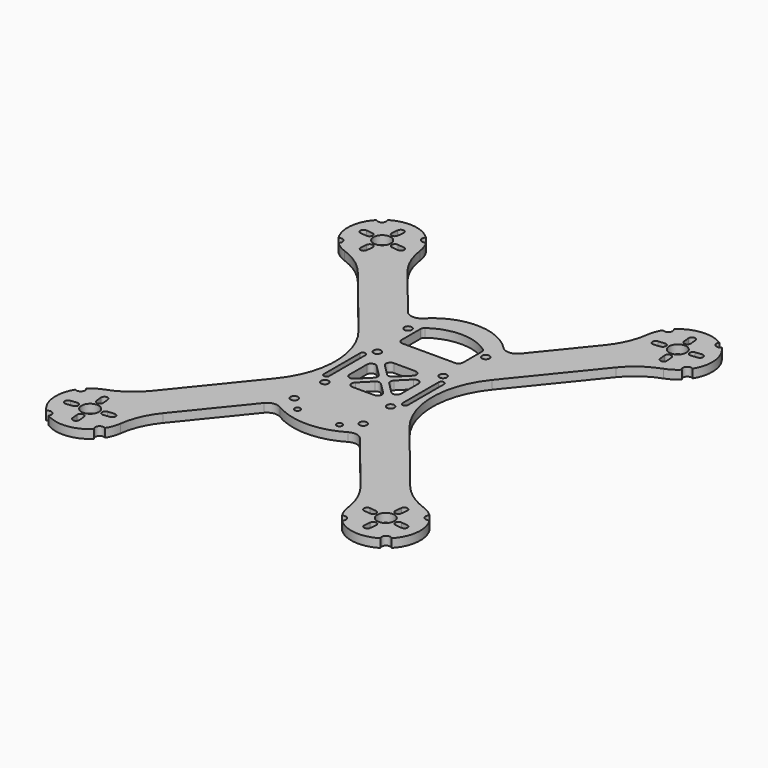
from build123d import *

# Parameters (mm, degrees)
F0_R     = 4
F0_R_2   = 1.35
F0_R_3   = 1.75
F1_DEPTH = 4
F3_DEPTH = 25


# Not quite as in the source:
# - a feature names something its author has since deleted; it is built from what else it names


with BuildPart() as f1:
    # F0 (on Top) → F1 (new body)
    with BuildSketch(Plane.XY):
        with BuildLine():
            ThreePointArc((59.8824194875, 59.6474879899), (66.2441988356, 65.6146941014), (73.980978501, 69.6423516913))
            ThreePointArc((73.980978501, 69.6423516913), (77.0154819314, 71.1033586862), (79.6769346686, 73.1671953648))
            ThreePointArc((79.6769346686, 73.1671953648), (79.4759660848, 75.8984243241), (82.1892948565, 76.269701817))
            ThreePointArc((82.1892948565, 76.269701817), (84.5082729503, 86.3813652111), (80.1376370585, 95.789921843))
            ThreePointArc((80.1376370585, 95.789921843), (77.4064080991, 95.5889532592), (77.0351306062, 98.3022820309))
            ThreePointArc((77.0351306062, 98.3022820309), (66.9234672121, 100.6212601247), (57.5149105803, 96.2506242328))
            ThreePointArc((57.5149105803, 96.2506242328), (57.715879164, 93.5193952735), (55.0025503923, 93.1481177806))
            ThreePointArc((55.0025503923, 93.1481177806), (53.5371606356, 90.1157283978), (52.7389888878, 86.8437757133))
            ThreePointArc((52.7389888878, 86.8437757133), (50.4079122214, 78.4386661467), (45.8937921813, 70.9752550288))
            Line((45.8937921813, 70.9752550288), (26.0751424851, 46.5012608726))
            ThreePointArc((26.0751424851, 46.5012608726), (22.420247462, 44.6531941399), (18.6104751491, 46.1562720492))
            ThreePointArc((18.6104751491, 46.1562720492), (0, 54), (-18.6104751491, 46.1562720492))
            ThreePointArc((-18.6104751491, 46.1562720492), (-22.420247462, 44.6531941399), (-26.0751424851, 46.5012608726))
            Line((-26.0751424851, 46.5012608726), (-45.8937921813, 70.9752550288))
            ThreePointArc((-45.8937921813, 70.9752550288), (-50.4079122214, 78.4386661467), (-52.7389888878, 86.8437757133))
            ThreePointArc((-52.7389888878, 86.8437757133), (-53.5371606356, 90.1157283978), (-55.0025503923, 93.1481177806))
            ThreePointArc((-55.0025503923, 93.1481177806), (-57.715879164, 93.5193952735), (-57.5149105803, 96.2506242328))
            ThreePointArc((-57.5149105803, 96.2506242328), (-66.9234672121, 100.6212601247), (-77.0351306062, 98.3022820309))
            ThreePointArc((-77.0351306062, 98.3022820309), (-77.4064080991, 95.5889532592), (-80.1376370585, 95.789921843))
            ThreePointArc((-80.1376370585, 95.789921843), (-84.5082729503, 86.3813652111), (-82.1892948565, 76.269701817))
            ThreePointArc((-82.1892948565, 76.269701817), (-79.4759660848, 75.8984243241), (-79.6769346686, 73.1671953648))
            ThreePointArc((-79.6769346686, 73.1671953648), (-77.0154819314, 71.1033586862), (-73.980978501, 69.6423516913))
            ThreePointArc((-73.980978501, 69.6423516913), (-66.2441988356, 65.6146941014), (-59.8824194875, 59.6474879899))
            Line((-59.8824194875, 59.6474879899), (-30.9461530616, 23.9141748599))
            ThreePointArc((-30.9461530616, 23.9141748599), (-22.477699597, 0), (-30.9461530616, -23.9141748599))
            Line((-30.9461530616, -23.9141748599), (-59.8824194875, -59.6474879899))
            ThreePointArc((-59.8824194875, -59.6474879899), (-66.2441988356, -65.6146941014), (-73.980978501, -69.6423516913))
            ThreePointArc((-73.980978501, -69.6423516913), (-77.0154819314, -71.1033586862), (-79.6769346686, -73.1671953648))
            ThreePointArc((-79.6769346686, -73.1671953648), (-79.4759660848, -75.8984243241), (-82.1892948565, -76.269701817))
            ThreePointArc((-82.1892948565, -76.269701817), (-84.5082729503, -86.3813652111), (-80.1376370585, -95.789921843))
            ThreePointArc((-80.1376370585, -95.789921843), (-77.4064080991, -95.5889532592), (-77.0351306062, -98.3022820309))
            ThreePointArc((-77.0351306062, -98.3022820309), (-66.9234672121, -100.6212601247), (-57.5149105803, -96.2506242328))
            ThreePointArc((-57.5149105803, -96.2506242328), (-57.715879164, -93.5193952735), (-55.0025503923, -93.1481177806))
            ThreePointArc((-55.0025503923, -93.1481177806), (-53.5371606356, -90.1157283978), (-52.7389888878, -86.8437757133))
            ThreePointArc((-52.7389888878, -86.8437757133), (-50.4079122214, -78.4386661467), (-45.8937921813, -70.9752550288))
            Line((-45.8937921813, -70.9752550288), (-22.2716253028, -41.8043083194))
            ThreePointArc((-22.2716253028, -41.8043083194), (-19.2665196055, -40.0290710679), (-15.8322988989, -40.6521727365))
            ThreePointArc((-15.8322988989, -40.6521727365), (0, -45), (15.8322988989, -40.6521727365))
            ThreePointArc((15.8322988989, -40.6521727365), (19.2665196055, -40.0290710679), (22.2716253028, -41.8043083194))
            Line((22.2716253028, -41.8043083194), (45.8937921813, -70.9752550288))
            ThreePointArc((45.8937921813, -70.9752550288), (50.4079122214, -78.4386661467), (52.7389888878, -86.8437757133))
            ThreePointArc((52.7389888878, -86.8437757133), (53.5371606356, -90.1157283978), (55.0025503923, -93.1481177806))
            ThreePointArc((55.0025503923, -93.1481177806), (57.715879164, -93.5193952735), (57.5149105803, -96.2506242328))
            ThreePointArc((57.5149105803, -96.2506242328), (66.9234672121, -100.6212601247), (77.0351306062, -98.3022820309))
            ThreePointArc((77.0351306062, -98.3022820309), (77.4064080991, -95.5889532592), (80.1376370585, -95.789921843))
            ThreePointArc((80.1376370585, -95.789921843), (84.5082729503, -86.3813652111), (82.1892948565, -76.269701817))
            ThreePointArc((82.1892948565, -76.269701817), (79.4759660848, -75.8984243241), (79.6769346686, -73.1671953648))
            ThreePointArc((79.6769346686, -73.1671953648), (77.0154819314, -71.1033586862), (73.980978501, -69.6423516913))
            ThreePointArc((73.980978501, -69.6423516913), (66.2441988356, -65.6146941014), (59.8824194875, -59.6474879899))
            Line((59.8824194875, -59.6474879899), (30.9461530616, -23.9141748599))
            ThreePointArc((30.9461530616, -23.9141748599), (22.477699597, 0), (30.9461530616, 23.9141748599))
            Line((30.9461530616, 23.9141748599), (59.8824194875, 59.6474879899))
        make_face()
        with BuildLine():
            Line((-69.0946850664, -94.3136604997), (-69.4082704562, -91.3300948136))
            ThreePointArc((-69.4082704562, -91.3300948136), (-68.0732803081, -89.6815192757), (-66.4247047701, -91.0165094238))
            Line((-66.4247047701, -91.0165094238), (-66.1111193803, -94.0000751099))
            ThreePointArc((-66.1111193803, -94.0000751099), (-67.4461095285, -95.6486506479), (-69.0946850664, -94.3136604997))
        make_face(mode=Mode.SUBTRACT)
        with BuildLine():
            Line((-78.2006733253, -84.2101473568), (-75.2171076392, -83.896561967))
            ThreePointArc((-75.2171076392, -83.896561967), (-73.5685321013, -85.2315521151), (-74.9035222494, -86.8801276531))
            Line((-74.9035222494, -86.8801276531), (-77.8870879355, -87.1937130429))
            ThreePointArc((-77.8870879355, -87.1937130429), (-79.5356634735, -85.8587228948), (-78.2006733253, -84.2101473568))
        make_face(mode=Mode.SUBTRACT)
        with Locations((-68.5959226244, -84.7089097988)):
            Circle(F0_R, mode=Mode.SUBTRACT)
        with BuildLine():
            ThreePointArc((-67.7835747926, -78.087724784), (-69.1185649408, -79.736300322), (-70.7671404787, -78.4013101738))
            Line((-70.7671404787, -78.4013101738), (-71.0807258685, -75.4177444877))
            ThreePointArc((-71.0807258685, -75.4177444877), (-69.7457357204, -73.7691689498), (-68.0971601824, -75.1041590979))
            Line((-68.0971601824, -75.1041590979), (-67.7835747926, -78.087724784))
        make_face(mode=Mode.SUBTRACT)
        with BuildLine():
            Line((-58.9911719235, -85.2076722408), (-61.9747376096, -85.5212576306))
            ThreePointArc((-61.9747376096, -85.5212576306), (-63.6233131476, -84.1862674825), (-62.2883229994, -82.5376919445))
            Line((-62.2883229994, -82.5376919445), (-59.3047573133, -82.2241065547))
            ThreePointArc((-59.3047573133, -82.2241065547), (-57.6561817754, -83.5590967029), (-58.9911719235, -85.2076722408))
        make_face(mode=Mode.SUBTRACT)
        with Locations((-9.75, -38)):
            Circle(F0_R_2, mode=Mode.SUBTRACT)
        with Locations((-16, -32)):
            Circle(F0_R_3, mode=Mode.SUBTRACT)
        with Locations((-15.25, -15.25)):
            Circle(F0_R_3, mode=Mode.SUBTRACT)
        with BuildLine():
            ThreePointArc((62.2883229994, -82.5376919445), (63.6233131476, -84.1862674825), (61.9747376096, -85.5212576306))
            Line((61.9747376096, -85.5212576306), (58.9911719235, -85.2076722408))
            ThreePointArc((58.9911719235, -85.2076722408), (57.6561817754, -83.5590967029), (59.3047573133, -82.2241065547))
            Line((59.3047573133, -82.2241065547), (62.2883229994, -82.5376919445))
        make_face(mode=Mode.SUBTRACT)
        with BuildLine():
            ThreePointArc((66.4247047701, -91.0165094238), (68.0732803081, -89.6815192757), (69.4082704562, -91.3300948136))
            Line((69.4082704562, -91.3300948136), (69.0946850664, -94.3136604997))
            ThreePointArc((69.0946850664, -94.3136604997), (67.4461095285, -95.6486506479), (66.1111193803, -94.0000751099))
            Line((66.1111193803, -94.0000751099), (66.4247047701, -91.0165094238))
        make_face(mode=Mode.SUBTRACT)
        with Locations((68.5959226244, -84.7089097988)):
            Circle(F0_R, mode=Mode.SUBTRACT)
        with BuildLine():
            ThreePointArc((70.7671404787, -78.4013101738), (69.1185649408, -79.736300322), (67.7835747926, -78.087724784))
            Line((67.7835747926, -78.087724784), (68.0971601824, -75.1041590979))
            ThreePointArc((68.0971601824, -75.1041590979), (69.7457357204, -73.7691689498), (71.0807258685, -75.4177444877))
            Line((71.0807258685, -75.4177444877), (70.7671404787, -78.4013101738))
        make_face(mode=Mode.SUBTRACT)
        with BuildLine():
            ThreePointArc((74.9035222494, -86.8801276531), (73.5685321013, -85.2315521151), (75.2171076392, -83.896561967))
            Line((75.2171076392, -83.896561967), (78.2006733253, -84.2101473568))
            ThreePointArc((78.2006733253, -84.2101473568), (79.5356634735, -85.8587228948), (77.8870879355, -87.1937130429))
            Line((77.8870879355, -87.1937130429), (74.9035222494, -86.8801276531))
        make_face(mode=Mode.SUBTRACT)
        with Locations((9.75, -38)):
            Circle(F0_R_2, mode=Mode.SUBTRACT)
        with Locations((16, -32)):
            Circle(F0_R_3, mode=Mode.SUBTRACT)
        with Locations((15.25, -15.25)):
            Circle(F0_R_3, mode=Mode.SUBTRACT)
        with BuildLine():
            Line((-19.5, -10.5), (-19.5, 10.5))
            ThreePointArc((-19.5, 10.5), (-18.25, 11.75), (-17, 10.5))
            Line((-17, 10.5), (-17, -10.5))
            ThreePointArc((-17, -10.5), (-18.25, -11.75), (-19.5, -10.5))
        make_face(mode=Mode.SUBTRACT)
        with Locations((-15.25, 15.25)):
            Circle(F0_R_3, mode=Mode.SUBTRACT)
        with Locations((-18, 36.5)):
            Circle(F0_R_3, mode=Mode.SUBTRACT)
        with BuildLine():
            Line((12.25, 26), (-12.25, 26))
            ThreePointArc((-12.25, 26), (-13.6642135624, 26.5857864376), (-14.25, 28))
            Line((-14.25, 28), (-14.25, 39.0031508785))
            ThreePointArc((-14.25, 39.0031508785), (-14.029513042, 39.9160218077), (-13.4166666667, 40.6276166027))
            ThreePointArc((-13.4166666667, 40.6276166027), (0, 44.9462607751), (13.4166666667, 40.6276166027))
            ThreePointArc((13.4166666667, 40.6276166027), (14.029513042, 39.9160218077), (14.25, 39.0031508785))
            Line((14.25, 39.0031508785), (14.25, 28))
            ThreePointArc((14.25, 28), (13.6642135624, 26.5857864376), (12.25, 26))
        make_face(mode=Mode.SUBTRACT)
        with BuildLine():
            ThreePointArc((-74.9035222494, 86.8801276531), (-73.5685321013, 85.2315521151), (-75.2171076392, 83.896561967))
            Line((-75.2171076392, 83.896561967), (-78.2006733253, 84.2101473568))
            ThreePointArc((-78.2006733253, 84.2101473568), (-79.5356634735, 85.8587228948), (-77.8870879355, 87.1937130429))
            Line((-77.8870879355, 87.1937130429), (-74.9035222494, 86.8801276531))
        make_face(mode=Mode.SUBTRACT)
        with BuildLine():
            ThreePointArc((-70.7671404787, 78.4013101738), (-69.1185649408, 79.736300322), (-67.7835747926, 78.087724784))
            Line((-67.7835747926, 78.087724784), (-68.0971601824, 75.1041590979))
            ThreePointArc((-68.0971601824, 75.1041590979), (-69.7457357204, 73.7691689498), (-71.0807258685, 75.4177444877))
            Line((-71.0807258685, 75.4177444877), (-70.7671404787, 78.4013101738))
        make_face(mode=Mode.SUBTRACT)
        with Locations((-68.5959226244, 84.7089097988)):
            Circle(F0_R, mode=Mode.SUBTRACT)
        with BuildLine():
            ThreePointArc((-66.4247047701, 91.0165094238), (-68.0732803081, 89.6815192757), (-69.4082704562, 91.3300948136))
            Line((-69.4082704562, 91.3300948136), (-69.0946850664, 94.3136604997))
            ThreePointArc((-69.0946850664, 94.3136604997), (-67.4461095285, 95.6486506479), (-66.1111193803, 94.0000751099))
            Line((-66.1111193803, 94.0000751099), (-66.4247047701, 91.0165094238))
        make_face(mode=Mode.SUBTRACT)
        with BuildLine():
            ThreePointArc((-62.2883229994, 82.5376919445), (-63.6233131476, 84.1862674825), (-61.9747376096, 85.5212576306))
            Line((-61.9747376096, 85.5212576306), (-58.9911719235, 85.2076722408))
            ThreePointArc((-58.9911719235, 85.2076722408), (-57.6561817754, 83.5590967029), (-59.3047573133, 82.2241065547))
            Line((-59.3047573133, 82.2241065547), (-62.2883229994, 82.5376919445))
        make_face(mode=Mode.SUBTRACT)
        with BuildLine():
            Line((19.5, 10.5), (19.5, -10.5))
            ThreePointArc((19.5, -10.5), (18.25, -11.75), (17, -10.5))
            Line((17, -10.5), (17, 10.5))
            ThreePointArc((17, 10.5), (18.25, 11.75), (19.5, 10.5))
        make_face(mode=Mode.SUBTRACT)
        with Locations((15.25, 15.25)):
            Circle(F0_R_3, mode=Mode.SUBTRACT)
        with Locations((18, 36.5)):
            Circle(F0_R_3, mode=Mode.SUBTRACT)
        with BuildLine():
            Line((62.2883229994, 82.5376919445), (59.3047573133, 82.2241065547))
            ThreePointArc((59.3047573133, 82.2241065547), (57.6561817754, 83.5590967029), (58.9911719235, 85.2076722408))
            Line((58.9911719235, 85.2076722408), (61.9747376096, 85.5212576306))
            ThreePointArc((61.9747376096, 85.5212576306), (63.6233131476, 84.1862674825), (62.2883229994, 82.5376919445))
        make_face(mode=Mode.SUBTRACT)
        with BuildLine():
            ThreePointArc((67.7835747926, 78.087724784), (69.1185649408, 79.736300322), (70.7671404787, 78.4013101738))
            Line((70.7671404787, 78.4013101738), (71.0807258685, 75.4177444877))
            ThreePointArc((71.0807258685, 75.4177444877), (69.7457357204, 73.7691689498), (68.0971601824, 75.1041590979))
            Line((68.0971601824, 75.1041590979), (67.7835747926, 78.087724784))
        make_face(mode=Mode.SUBTRACT)
        with Locations((68.5959226244, 84.7089097988)):
            Circle(F0_R, mode=Mode.SUBTRACT)
        with BuildLine():
            Line((78.2006733253, 84.2101473568), (75.2171076392, 83.896561967))
            ThreePointArc((75.2171076392, 83.896561967), (73.5685321013, 85.2315521151), (74.9035222494, 86.8801276531))
            Line((74.9035222494, 86.8801276531), (77.8870879355, 87.1937130429))
            ThreePointArc((77.8870879355, 87.1937130429), (79.5356634735, 85.8587228948), (78.2006733253, 84.2101473568))
        make_face(mode=Mode.SUBTRACT)
        with BuildLine():
            ThreePointArc((69.4082704562, 91.3300948136), (68.0732803081, 89.6815192757), (66.4247047701, 91.0165094238))
            Line((66.4247047701, 91.0165094238), (66.1111193803, 94.0000751099))
            ThreePointArc((66.1111193803, 94.0000751099), (67.4461095285, 95.6486506479), (69.0946850664, 94.3136604997))
            Line((69.0946850664, 94.3136604997), (69.4082704562, 91.3300948136))
        make_face(mode=Mode.SUBTRACT)
    extrude(amount=F1_DEPTH)

    # F2 (on face) → F3 (cut)
    with BuildSketch(Plane.XY.offset(4)):
        with BuildLine():
            Line((5.0502525317, 12), (-5.0502525317, 12))
            ThreePointArc((-5.0502525317, 12), (-6.8980115967, 10.7653668647), (-6.4644660941, 8.5857864376))
            Line((-6.4644660941, 8.5857864376), (-1.4142135624, 3.5355339059))
            ThreePointArc((-1.4142135624, 3.5355339059), (0, 2.9497474683), (1.4142135624, 3.5355339059))
            Line((1.4142135624, 3.5355339059), (6.4644660941, 8.5857864376))
            ThreePointArc((6.4644660941, 8.5857864376), (6.8980115967, 10.7653668647), (5.0502525317, 12))
        make_face()
        with BuildLine():
            ThreePointArc((-6.4644660941, -8.5857864376), (-6.8980115967, -10.7653668647), (-5.0502525317, -12))
            Line((-5.0502525317, -12), (5.0502525317, -12))
            ThreePointArc((5.0502525317, -12), (6.8980115967, -10.7653668647), (6.4644660941, -8.5857864376))
            Line((6.4644660941, -8.5857864376), (1.4142135624, -3.5355339059))
            ThreePointArc((1.4142135624, -3.5355339059), (0, -2.9497474683), (-1.4142135624, -3.5355339059))
            Line((-1.4142135624, -3.5355339059), (-6.4644660941, -8.5857864376))
        make_face()
        with BuildLine():
            ThreePointArc((-8.5857864376, 6.4644660941), (-10.7653668647, 6.8980115967), (-12, 5.0502525317))
            Line((-12, 5.0502525317), (-12, -5.0502525317))
            ThreePointArc((-12, -5.0502525317), (-10.7653668647, -6.8980115967), (-8.5857864376, -6.4644660941))
            Line((-8.5857864376, -6.4644660941), (-3.5355339059, -1.4142135624))
            ThreePointArc((-3.5355339059, -1.4142135624), (-2.9497474683, 0), (-3.5355339059, 1.4142135624))
            Line((-3.5355339059, 1.4142135624), (-8.5857864376, 6.4644660941))
        make_face()
        with BuildLine():
            Line((12, -5.0502525317), (12, 5.0502525317))
            ThreePointArc((12, 5.0502525317), (10.7653668647, 6.8980115967), (8.5857864376, 6.4644660941))
            Line((8.5857864376, 6.4644660941), (3.5355339059, 1.4142135624))
            ThreePointArc((3.5355339059, 1.4142135624), (2.9497474683, 0), (3.5355339059, -1.4142135624))
            Line((3.5355339059, -1.4142135624), (8.5857864376, -6.4644660941))
            ThreePointArc((8.5857864376, -6.4644660941), (10.7653668647, -6.8980115967), (12, -5.0502525317))
        make_face()
    extrude(amount=-F3_DEPTH, mode=Mode.SUBTRACT)


solid = f1.part
